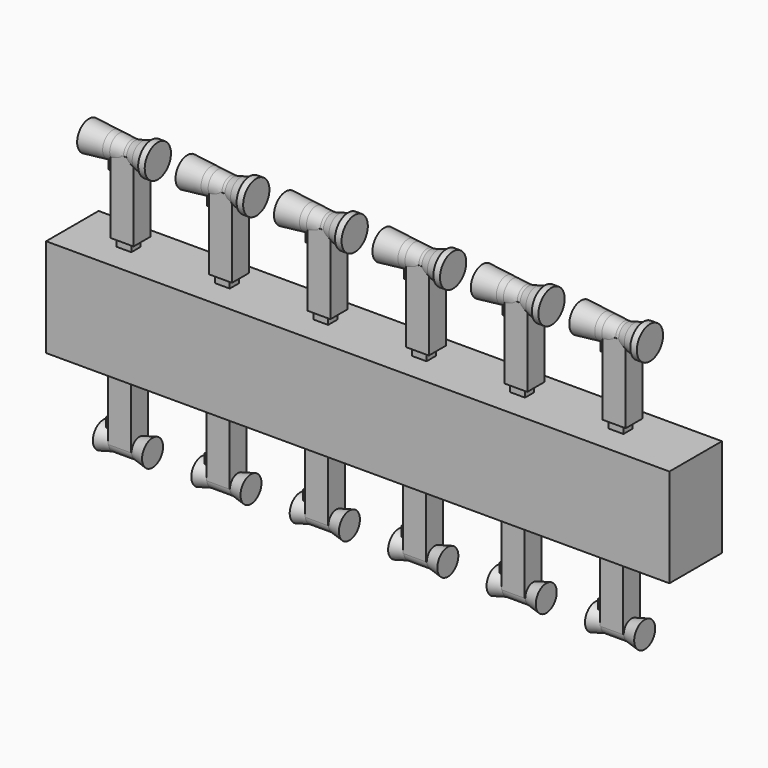
from build123d import *

# Parameters (mm, degrees)
F0_W     = 0.2
F0_H     = 0.32
F0_W_2   = 0.2197528529
F2_DEPTH = 0.15
F3_DEPTH = 0.325
F0_W_3   = 0.7
F0_H_2   = 0.3
F5_DEPTH = 0.325
F6_DEPTH = 0.15
F0_W_4   = 0.45
F0_H_3   = 0.2867222825
F0_H_4   = 0.0132777175
F7_DEPTH = 0.175
F0_H_5   = 0.2767520538
F0_H_6   = 0.0232479462
F8_DEPTH = 0.175
F9_DEPTH = 1


with BuildPart() as f1:
    # F0 (on Front) → F1 (revolve)
    with BuildSketch(Plane.XZ):
        with Locations((-0.5802471471, 0.16)):
            Rectangle(F0_W, F0_H)
        Polygon((-0.4802471471, -0.0386663069), (-0.4802471471, 0), (-0.6802471471, 0), (-0.6802471471, -0.0585267928), align=None)
        Polygon((-0.0908678849, 0), (-0.4802471471, 0), (-0.4802471471, -0.0386663069), align=None)
        Polygon((-0.4802471471, 0.32), (-0.4802471471, 0), (-0.0908678849, 0), (0, 0), (0, 0.32), align=None)
        with Locations((0.1098764264, 0.16)):
            Rectangle(F0_W_2, F0_H)
        Polygon((0.2197528529, 0), (0, 0), (0.2197528529, -0.0571357417), align=None)
        Polygon((0.5, 0.32), (0.5, -0.13), (0.5, -0.18), (0.7, -0.18), (0.7, 0.32), align=None)
        Polygon((0.2197528529, 0.32), (0.2197528529, 0), (0.2197528529, -0.0571357417), (0.5, -0.13), (0.5, 0.32), align=None)
        Polygon((-0.6802471471, -0.0585267928), (-0.6802471471, 0), (-0.6802471471, 0.32), (-1.4, 0.32), (-1.4, -0.13), align=None)
    revolve(axis=Axis((-0.7, 0, 0.32), (1, 0, 0)))

    # F0 (on Front) → F2 (join, symmetric)
    with BuildSketch(Plane.XZ):
        Polygon((-0.4802471471, -0.3), (-0.4802471471, -0.0386663069), (-0.6802471471, -0.0585267928), (-0.6802471471, -0.3), align=None)
        with Locations((-0.5802471471, 0.16)):
            Rectangle(F0_W, F0_H)
        Polygon((-0.4802471471, -0.0386663069), (-0.4802471471, 0), (-0.6802471471, 0), (-0.6802471471, -0.0585267928), align=None)
    extrude(amount=F2_DEPTH, both=True)

    # F0 (on Front) → F3 (join, symmetric)
    with BuildSketch(Plane.XZ):
        Polygon((0, 0), (-0.0908678849, 0), (-0.4802471471, -0.0386663069), (-0.4802471471, -0.3), (-0.4802471471, -2), (-0.4187109589, -2), (0.0312890411, -2), (0.2197528529, -2), (0.2197528529, -0.0571357417), align=None)
        Polygon((-0.0908678849, 0), (-0.4802471471, 0), (-0.4802471471, -0.0386663069), align=None)
        Polygon((0.2197528529, 0), (0, 0), (0.2197528529, -0.0571357417), align=None)
        Polygon((-0.4802471471, 0.32), (-0.4802471471, 0), (-0.0908678849, 0), (0, 0), (0, 0.32), align=None)
        with Locations((0.1098764264, 0.16)):
            Rectangle(F0_W_2, F0_H)
    extrude(amount=F3_DEPTH, both=True)

    # F0 (on Front) → F8 (join, symmetric)
    with BuildSketch(Plane.XZ):
        with Locations((-0.1937109589, -2.1383760269)):
            Rectangle(F0_W_4, F0_H_5)
        with Locations((-0.1937109589, -2.2883760269)):
            Rectangle(F0_W_4, F0_H_6)
    extrude(amount=F8_DEPTH, both=True)


with BuildPart() as f4:
    # F0 (on Front) → F4 (revolve)
    with BuildSketch(Plane.XZ):
        Polygon((0.5390828506, -7.1634743363), (0.1390828506, -7.2634743363), (0.1390828506, -7.5634743363), (0.5390828506, -7.5634743363), align=None)
        Polygon((-0.5609171494, -7.5634743363), (-0.5609171494, -7.2634743363), (-0.7609171494, -7.2134743363), (-0.7609171494, -7.5634743363), align=None)
        Polygon((-0.7609171494, -7.5634743363), (-0.7609171494, -7.2134743363), (-0.9609171494, -7.1634743363), (-0.9609171494, -7.5634743363), align=None)
        with Locations((-0.2109171494, -7.4134743363)):
            Rectangle(F0_W_3, F0_H_2)
    revolve(axis=Axis((0.3390828506, 0, -7.5634743363), (1, 0, 0)))

    # F0 (on Front) → F5 (join, symmetric)
    with BuildSketch(Plane.XZ):
        Polygon((-0.45, -5.5767520538), (-0.45, -5.5634743363), (-0.5609171494, -5.5634743363), (-0.5609171494, -6.9634743363), (-0.5609171494, -7.2634743363), (0.1390828506, -7.2634743363), (0.1390828506, -5.5634743363), (0, -5.5634743363), (0, -5.5767520538), align=None)
        with Locations((-0.2109171494, -7.4134743363)):
            Rectangle(F0_W_3, F0_H_2)
    extrude(amount=F5_DEPTH, both=True)

    # F0 (on Front) → F6 (join, symmetric)
    with BuildSketch(Plane.XZ):
        Polygon((-0.5609171494, -7.2634743363), (-0.5609171494, -6.9634743363), (-0.7609171494, -6.9634743363), (-0.7609171494, -7.2134743363), align=None)
        Polygon((-0.5609171494, -7.5634743363), (-0.5609171494, -7.2634743363), (-0.7609171494, -7.2134743363), (-0.7609171494, -7.5634743363), align=None)
    extrude(amount=F6_DEPTH, both=True)

    # F0 (on Front) → F7 (join, symmetric)
    with BuildSketch(Plane.XZ):
        with Locations((-0.225, -5.420113195)):
            Rectangle(F0_W_4, F0_H_3)
        with Locations((-0.225, -5.570113195)):
            Rectangle(F0_W_4, F0_H_4)
    extrude(amount=F7_DEPTH, both=True)


with BuildPart() as f9:
    # F0 (on Front) → F9 (new body, symmetric)
    with BuildSketch(Plane.XZ):
        Polygon((-0.4187109589, -2.3), (-0.4187109589, -2.2767520538), (-4.9067612272, -2.2767520538), (-4.9067612272, -5.2767520538), (-0.45, -5.2767520538), (0, -5.2767520538), (14.0932387728, -5.2767520538), (14.0932387728, -2.2767520538), (0.0312890411, -2.2767520538), (0.0312890411, -2.3), align=None)
        with Locations((-0.1937109589, -2.2883760269)):
            Rectangle(F0_W_4, F0_H_6)
    extrude(amount=F9_DEPTH, both=True)


with BuildPart() as f10_1:
    # F10: copy of F4
    add(f4.part.moved(Location((3, 0, 0))))


with BuildPart() as f11_1:
    # F11: copy of F4
    add(f4.part.moved(Location((-3, 0, 0))))


with BuildPart() as f12_1:
    # F12: copy of F1
    add(f1.part.moved(Location((3, 0, 0))))


with BuildPart() as f13_1:
    # F13: copy of F1
    add(f1.part.moved(Location((-3, 0, 0))))


with BuildPart() as f14_1:
    # F14: copy of F4
    add(f4.part.moved(Location((6, 0, 0))))


with BuildPart() as f15_1:
    # F15: copy of F4
    add(f4.part.moved(Location((9, 0, 0))))


with BuildPart() as f16_1:
    # F16: copy of F4
    add(f4.part.moved(Location((12, 0, 0))))


with BuildPart() as f17_1:
    # F17: copy of F1
    add(f1.part.moved(Location((6, 0, 0))))


with BuildPart() as f18_1:
    # F18: copy of F1
    add(f1.part.moved(Location((12, 0, 0))))


with BuildPart() as f19_1:
    # F19: copy of F1
    add(f1.part.moved(Location((9, 0, 0))))


solid = Compound([f1.part, f4.part, f9.part, f10_1.part, f11_1.part, f12_1.part, f13_1.part, f14_1.part, f15_1.part, f16_1.part, f17_1.part, f18_1.part, f19_1.part])
